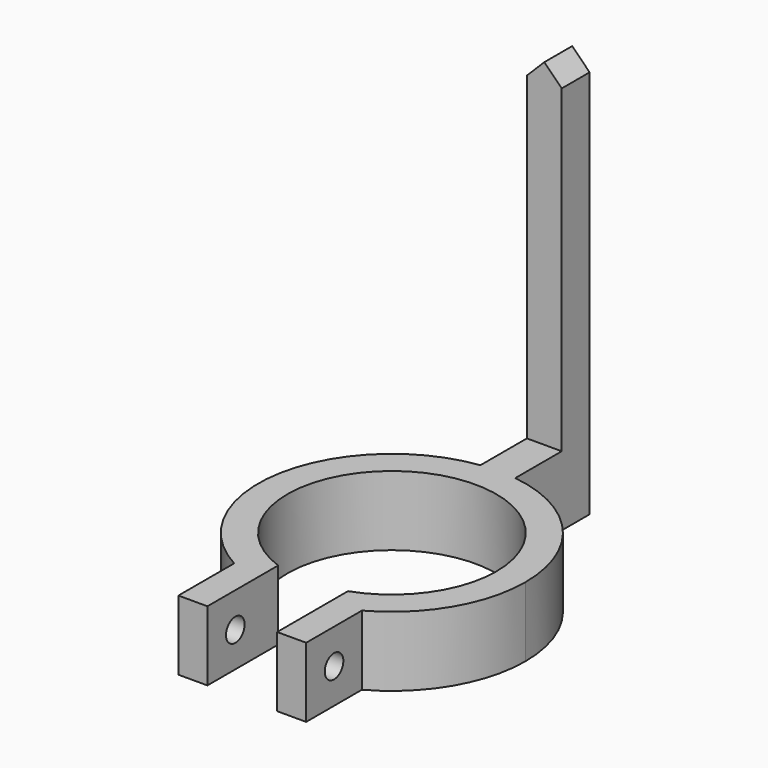
from build123d import *

# Parameters (mm, degrees)
F1_DEPTH = 6
F2_W     = 3
F2_H     = 3
F3_DEPTH = 29
F5_D     = 2
F6_SIZE  = 1.49999


# Not quite as in the source:
# - a fillet or chamfer is up to 0.001 mm smaller than in the source, because OpenCascade refuses the exact size


with BuildPart() as f1:
    # F0 (on Top) → F1 (new body)
    with BuildSketch(Plane.XY):
        with BuildLine():
            ThreePointArc((-3, -8.4852813742), (-5.1961524227, 7.3484692283), (9, 0))
            ThreePointArc((9, 0), (7.3484692283, -5.1961524227), (3, -8.4852813742))
            Line((3, -8.4852813742), (3, -11.1018016556))
            ThreePointArc((3, -11.1018016556), (4.2794450198, -10.6740971666), (5.5, -10.0995049384))
            ThreePointArc((5.5, -10.0995049384), (9.8868599666, -5.8736700622), (11.5, 0))
            ThreePointArc((11.5, 0), (8.6458082329, 7.5828754441), (1.5, 11.401754251))
            ThreePointArc((1.5, 11.401754251), (0, 11.5), (-1.5, 11.401754251))
            ThreePointArc((-1.5, 11.401754251), (-11.3060177199, 2.103321972), (-5.5, -10.0995049384))
            ThreePointArc((-5.5, -10.0995049384), (-4.2794450198, -10.6740971666), (-3, -11.1018016556))
            Line((-3, -11.1018016556), (-3, -8.4852813742))
        make_face()
        with BuildLine():
            ThreePointArc((5.5, -10.0995049384), (4.2794450198, -10.6740971666), (3, -11.1018016556))
            Line((3, -11.1018016556), (3, -16.0995049384))
            Line((3, -16.0995049384), (5.5, -16.0995049384))
            Line((5.5, -16.0995049384), (5.5, -10.0995049384))
        make_face()
        with BuildLine():
            Line((-3, -16.0995049384), (-3, -11.1018016556))
            ThreePointArc((-3, -11.1018016556), (-4.2794450198, -10.6740971666), (-5.5, -10.0995049384))
            Line((-5.5, -10.0995049384), (-5.5, -16.0995049384))
            Line((-5.5, -16.0995049384), (-3, -16.0995049384))
        make_face()
        with BuildLine():
            Line((-1.5, 19.401754251), (-1.5, 11.401754251))
            ThreePointArc((-1.5, 11.401754251), (0, 11.5), (1.5, 11.401754251))
            Line((1.5, 11.401754251), (1.5, 19.401754251))
            Line((1.5, 19.401754251), (-1.5, 19.401754251))
        make_face()
    extrude(amount=F1_DEPTH)

    # F2 (on face) → F3 (join)
    with BuildSketch(Plane.XY.offset(6)):
        with Locations((0, 17.901754251)):
            Rectangle(F2_W, F2_H)
    extrude(amount=F3_DEPTH)

    # F5 (through all)
    with Locations(Plane(origin=(-5.5, 0, 0), x_dir=(0, -1, 0), z_dir=(-1, 0, 0))):
        with Locations((13.0995049384, 3)):
            Hole(F5_D / 2)

    # F6 (size 1.5 in the source; OpenCascade refuses exactly that, so slightly less here)
    f6_edges = [f1.edges().sort_by_distance(p)[0] for p in [
        (1.5, 17.901754, 35),
        (-1.5, 17.901754, 35),
    ]]
    chamfer(f6_edges, length=F6_SIZE)


solid = f1.part
